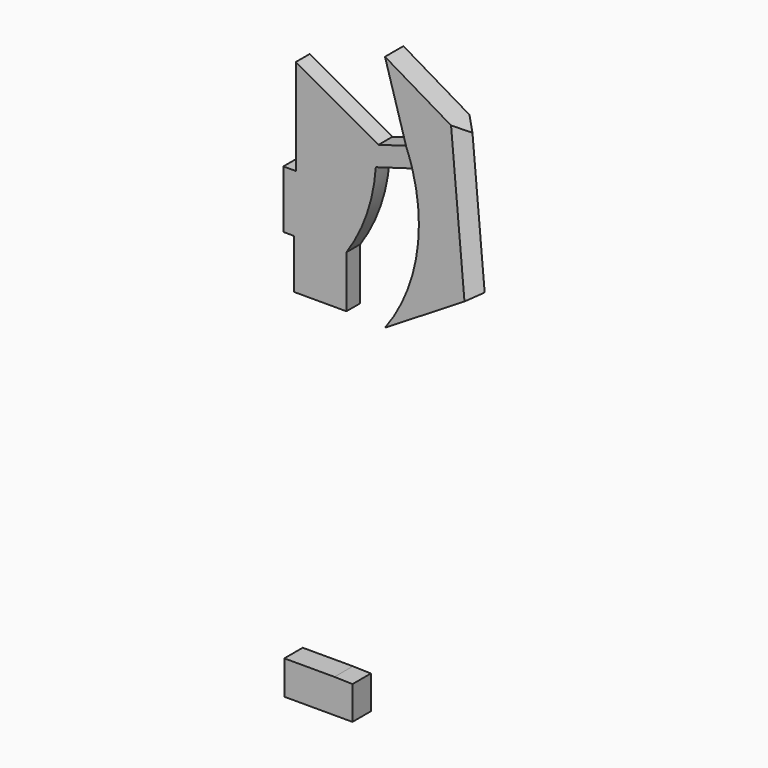
from build123d import *

# Parameters (mm, degrees)
F3_DEPTH    = 1.905
F4_DEPTH    = 2.54
F5_T1_DEPTH = 48.3053442814
F6_DEPTH    = 2.54


# Not quite as in the source:
# - a fillet or chamfer that OpenCascade refuses, or shapes differently, is made with other operations: its cross-section is extruded or revolved along the edge and cut away or added
# - the program builds the solid bodies; features that only make, move or delete a surface that nothing else refers to are left out


with BuildPart() as f3:
    # F0 (on Front) → F3 (new body, symmetric)
    with BuildSketch(Plane.XZ):
        with BuildLine():
            Line((-1.9319759193, 34.6202871443), (-20.1738812029, 44.7546765208))
            Line((-20.1738812029, 44.7546765208), (-20.1738812029, 23.6014798284))
            Line((-20.1738812029, 23.6014798284), (-22.9159612209, 23.6014798284))
            Line((-22.9159612209, 23.6014798284), (-22.9159612209, 10.8703924343))
            Line((-22.9159612209, 10.8703924343), (-20.5656066537, 10.8703924343))
            Line((-20.5656066537, 10.8703924343), (-20.5656066537, 0))
            Line((-20.5656066537, 0), (-18.231138587, 0))
            Line((-18.231138587, 0), (-14.9366050027, 0))
            Line((-14.9366050027, 0), (-11.6420714185, 0))
            Line((-11.6420714185, 0), (-11.3464937492, 0))
            Line((-11.3464937492, 0), (-9.0096937492, 0))
            Line((-9.0096937492, 0), (-9.0096937492, 11.4579806104))
            ThreePointArc((-9.0096937492, 11.4579806104), (-4.5198612968, 20.3362668162), (-2.5268969009, 30.0836077008))
            Line((-2.5268969009, 30.0836077008), (6.0717510059, 32.6111763716))
            ThreePointArc((6.0717510059, 32.6111763716), (5.4469320969, 34.6111548057), (4.7112164165, 36.5730505327))
            Line((4.7112164165, 36.5730505327), (-1.9319759193, 34.6202871443))
        make_face()
    extrude(amount=F3_DEPTH, both=True)

    # F0 (on Front) → F4 (join, symmetric)
    with BuildSketch(Plane.XZ):
        with BuildLine():
            Line((0, 52.6003465056), (4.7112164165, 36.5730505327))
            ThreePointArc((4.7112164165, 36.5730505327), (5.4469320969, 34.6111548057), (6.0717510059, 32.6111763716))
            ThreePointArc((6.0717510059, 32.6111763716), (6.8442642331, 15.59651876), (0, 0))
            Line((0, 0), (21.1531929672, 13.0248842761))
            Line((21.1531929672, 13.0248842761), (18.6069775373, 41.6208691895))
            Line((18.6069775373, 41.6208691895), (0, 52.6003465056))
        make_face()
    extrude(amount=F4_DEPTH, both=True)

    # F5: chamfer of 3.81 on 2 edges, made by hand

    # F5_s2 → F5_t1 (cut)
    with BuildSketch(Plane(origin=(-0.1152408587, 0, 1.2942447122), x_dir=(0, 1, 0), z_dir=(-0.0886901249, 0, 0.9960592662))):
        Polygon((-2.54, -18.4150124772), (1.27, -22.2250124772), (-2.54, -22.2250124772), align=None)
        Polygon((2.54, -18.4150124772), (-1.27, -22.2250124772), (2.54, -22.2250124772), align=None)
    extrude(amount=F5_T1_DEPTH, mode=Mode.SUBTRACT)


with BuildPart() as f6:
    # F0 (on Front) → F6 (new body, symmetric)
    with BuildSketch(Plane.XZ):
        Polygon((-14.7427194752, -78.8446590304), (-14.7427194752, -71.3911727071), (-18.3530040085, -71.3911727071), (-22.1962090582, -71.3911727071), (-22.1962090582, -78.8446590304), align=None)
        Polygon((-11.1324349418, -71.3911727071), (-14.7427194752, -71.3911727071), (-14.7427194752, -78.8446590304), (-7.1727680042, -78.8446590304), (-7.1727680042, -71.5076327324), align=None)
    extrude(amount=F6_DEPTH, both=True)


solid = Compound([f3.part, f6.part])
